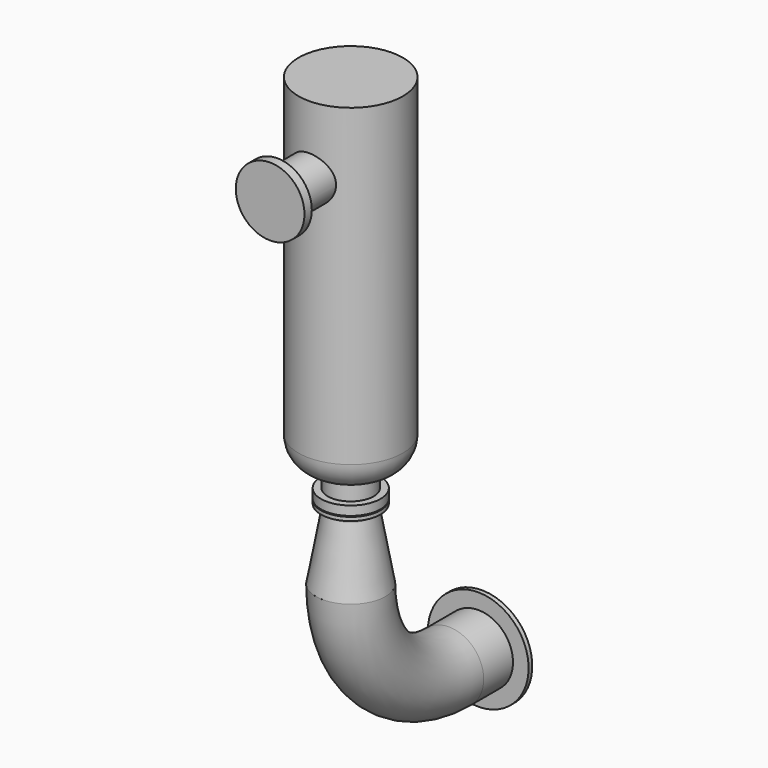
from build123d import *

# Parameters (mm, degrees)
F0_R      = 57
F1_DEPTH  = 375
F2_R      = 32
F3_R      = 25
F4_DEPTH  = 110
F5_R      = 37.5
F5_R_2    = 25
F6_DEPTH  = 10
F7_R      = 25
F8_DEPTH  = 30
F9_R      = 32.5
F9_R_2    = 25
F10_DEPTH = 10
F12_R     = 25
F13_DEPTH = 9
F14_R     = 32.5
F14_R_2   = 25
F15_DEPTH = 4
F18_R     = 38
F19_ANGLE = 90
F20_R     = 38
F21_DEPTH = 45
F22_R     = 55
F22_R_2   = 38
F23_DEPTH = 5


with BuildPart() as f1:
    # F0 (on Top) → F1 (new body)
    with BuildSketch(Plane.XY):
        Circle(F0_R)
    extrude(amount=F1_DEPTH)

    # F2
    f2_edges = [f1.edges().sort_by_distance(p)[0] for p in [
        (-57, 0, 0),
    ]]
    fillet(f2_edges, radius=F2_R)

    # F3 (on Front) → F4 (join)
    with BuildSketch(Plane.XZ):
        with Locations((0, 300)):
            Circle(F3_R)
    extrude(amount=F4_DEPTH)

    # F5 (on face) → F6 (join)
    with BuildSketch(Plane.XZ.offset(110)):
        with Locations((0, 300)):
            Circle(F5_R)
        with Locations((0, 300)):
            Circle(F5_R_2, mode=Mode.SUBTRACT)
    extrude(amount=-F6_DEPTH)

    # F7 (on face) → F8 (join)
    with BuildSketch(Plane(origin=(0, 0, 0), x_dir=(1, 0, 0), z_dir=(0, 0, -1))):
        Circle(F7_R)
    extrude(amount=F8_DEPTH)

    # F9 (on face) → F10 (join)
    with BuildSketch(Plane(origin=(0, 0, -30), x_dir=(1, 0, 0), z_dir=(0, 0, -1))):
        Circle(F9_R)
        Circle(F9_R_2, mode=Mode.SUBTRACT)
    extrude(amount=-F10_DEPTH)


with BuildPart() as f13:
    # F12 (on offset) → F13 (new body)
    with BuildSketch(Plane(origin=(0, 0, -31), x_dir=(1, 0, 0), z_dir=(0, 0, -1))):
        Circle(F12_R)
    extrude(amount=F13_DEPTH)

    # F14 (on face) → F15 (join)
    with BuildSketch(Plane.XY.offset(-31)):
        Circle(F14_R)
        Circle(F14_R_2, mode=Mode.SUBTRACT)
    extrude(amount=-F15_DEPTH)

    # F16 (on Front) → F17 (revolve)
    with BuildSketch(Plane.XZ):
        Polygon((0, -112), (0, -40), (-25, -40), (-38, -112), align=None)
    revolve(axis=Axis((0, 0, -76), (0, 0, -1)))


with BuildPart() as f19:
    # F18 (on face) → F19 (revolve)
    with BuildSketch(Plane(origin=(0, 0, -112), x_dir=(1, 0, 0), z_dir=(0, 0, -1))):
        Circle(F18_R)
    revolve(axis=Axis((-15.2300149202, 134, -112), (1, 0, 0)), revolution_arc=F19_ANGLE)

    # F20 (on face) → F21 (join)
    with BuildSketch(Plane(origin=(0, 134, 0), x_dir=(-1, 0, 0), z_dir=(0, 1, 0))):
        with Locations((0, -246)):
            Circle(F20_R)
    extrude(amount=F21_DEPTH)


with BuildPart() as f23:
    # F22 (on face) → F23 (new body)
    with BuildSketch(Plane(origin=(0, 179, 0), x_dir=(-1, 0, 0), z_dir=(0, 1, 0))):
        with Locations((0, -246)):
            Circle(F22_R)
        with Locations((0, -246)):
            Circle(F22_R_2, mode=Mode.SUBTRACT)
    extrude(amount=-F23_DEPTH)


solid = Compound([f1.part, f13.part, f19.part, f23.part])
